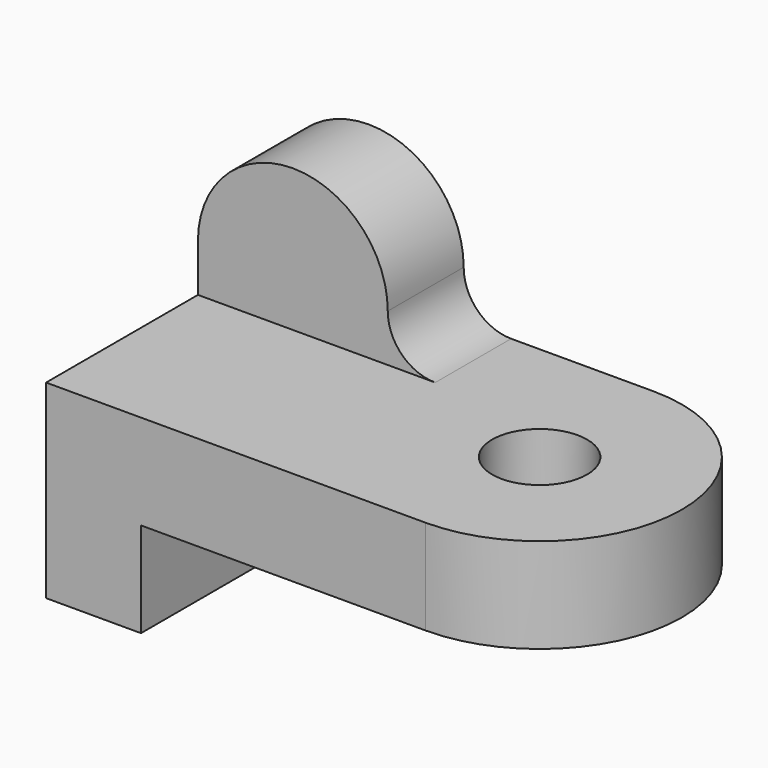
from build123d import *

# Parameters (mm, degrees)
F0_R     = 6.35
F0_W     = 12.7
F0_H     = 38.1
F1_DEPTH = 12.7
F2_DEPTH = 12.7
F4_DEPTH = 12.7


# Not quite as in the source:
# - a feature names something its author has since deleted; it is built from what else it names


with BuildPart() as f1:
    # F0 (on Top) → F1 (new body)
    with BuildSketch(Plane.XY):
        with BuildLine():
            Line((38.1, 0), (0, 0))
            Line((0, 0), (0, -38.1))
            Line((0, -38.1), (38.1, -38.1))
            ThreePointArc((38.1, -38.1), (57.15, -19.05), (38.1, 0))
        make_face()
        with Locations((38.1, -19.05)):
            Circle(F0_R, mode=Mode.SUBTRACT)
        with Locations((-6.35, -19.05)):
            Rectangle(F0_W, F0_H)
    extrude(amount=F1_DEPTH)

    # F0 (on Top) → F2 (join)
    with BuildSketch(Plane.XY):
        with Locations((-6.35, -19.05)):
            Rectangle(F0_W, F0_H)
    extrude(amount=-F2_DEPTH)

    # F3 (on face) → F4 (join)
    with BuildSketch(Plane(origin=(0, 0, 0), x_dir=(-1, 0, 0), z_dir=(0, 1, 0))):
        with BuildLine():
            Line((-19.05, 12.7), (12.7, 12.7))
            Line((12.7, 12.7), (12.7, 19.05))
            ThreePointArc((12.7, 19.05), (0, 31.75), (-12.7, 19.05))
            ThreePointArc((-12.7, 19.05), (-14.5598719395, 14.5598719395), (-19.05, 12.7))
        make_face()
    extrude(amount=-F4_DEPTH)


solid = f1.part
